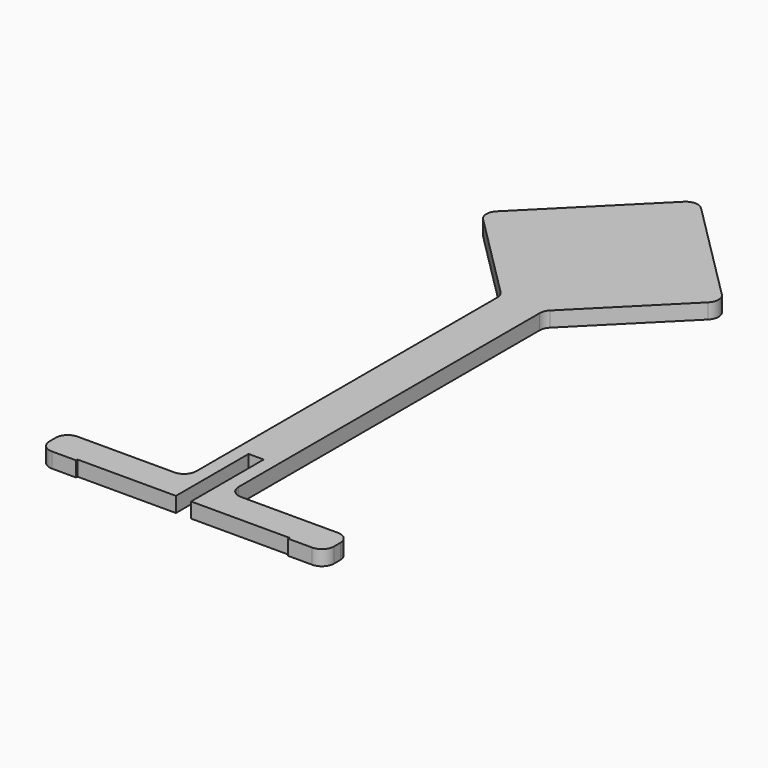
from build123d import *

# Parameters (mm, degrees)
F0_W     = 6
F0_H     = 0.3
F1_DEPTH = 2.5
F2_R     = 2


# Not quite as in the source:
# - a feature names something its author has since deleted; it is built from what else it names


with BuildPart() as f1:
    # F0 (on Top) → F1 (new body)
    with BuildSketch(Plane.XY):
        Polygon((0, -4), (-3.5, -0.5), (-3.5, -65.5), (-23.5, -65.5), (-23.5, -70.5), (-17.5, -70.5), (-1.25, -70.5), (-1.25, -55.5), (1.25, -55.5), (1.25, -70.5), (17.5, -70.5), (23.5, -70.5), (23.5, -65.5), (3.5, -65.5), (3.5, -0.5), align=None)
        with Locations((-20.5, -70.65)):
            Rectangle(F0_W, F0_H)
        with Locations((20.5, -70.65)):
            Rectangle(F0_W, F0_H)
        Polygon((-20, 16), (-3.5, -0.5), (0, -4), (3.5, -0.5), (20, 16), (0, 36), align=None)
    extrude(amount=F1_DEPTH)

    # F2
    f2_edges = [f1.edges().sort_by_distance(p)[0] for p in [
        (3.5, -65.5, 1.25),
        (-3.5, -65.5, 1.25),
        (-23.5, -65.5, 1.25),
        (23.5, -65.5, 1.25),
        (-23.5, -70.8, 1.25),
        (23.5, -70.8, 1.25),
        (20, 16, 1.25),
        (0, 36, 1.25),
        (-20, 16, 1.25),
        (3.5, -0.5, 1.25),
        (-3.5, -0.5, 1.25),
    ]]
    fillet(f2_edges, radius=F2_R)


solid = f1.part
